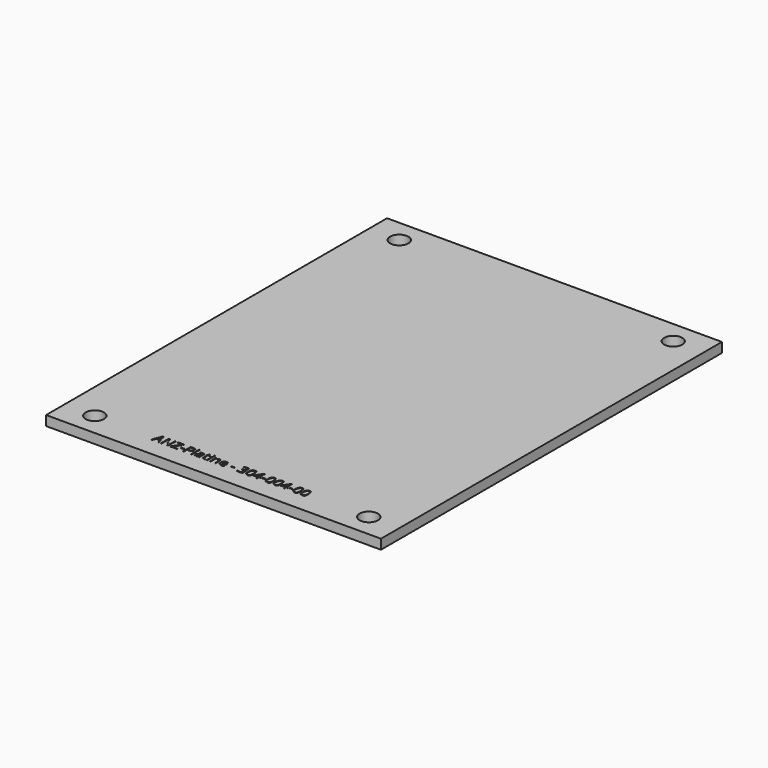
from build123d import *

# Parameters (mm, degrees)
F0_W         = 55
F0_H         = 70
F0_R         = 1.5
F1_DEPTH     = 1.6
F2_TEXT_SIZE = 2.2051416131
F3_DEPTH     = 0.1


# Not quite as in the source:
# - Text() gives the source's letters only with a copy of the font that has no kerning and outlines rounded to 1/6400 em; it was checked with that copy


with BuildPart() as f1:
    # F0 (on Top) → F1 (new body)
    with BuildSketch(Plane.XY):
        Rectangle(F0_W, F0_H)
        with Locations((-22.5, -31.25)):
            Circle(F0_R, mode=Mode.SUBTRACT)
        with Locations((22.5, -31.25)):
            Circle(F0_R, mode=Mode.SUBTRACT)
        with Locations((-22.5, 31.25)):
            Circle(F0_R, mode=Mode.SUBTRACT)
        with Locations((22.5, 31.25)):
            Circle(F0_R, mode=Mode.SUBTRACT)
    extrude(amount=-F1_DEPTH)

    # F2 (on face) → F3 (cut)
    with BuildSketch(Plane.XY):
        with Locations((-12.7221322618, -31.9066271186)):
            Text('ANZ-Platine - 304-004-00', F2_TEXT_SIZE, font='Open Sans', text_align=(TextAlign.LEFT, TextAlign.BOTTOM))
    extrude(amount=-F3_DEPTH, mode=Mode.SUBTRACT)


solid = f1.part
